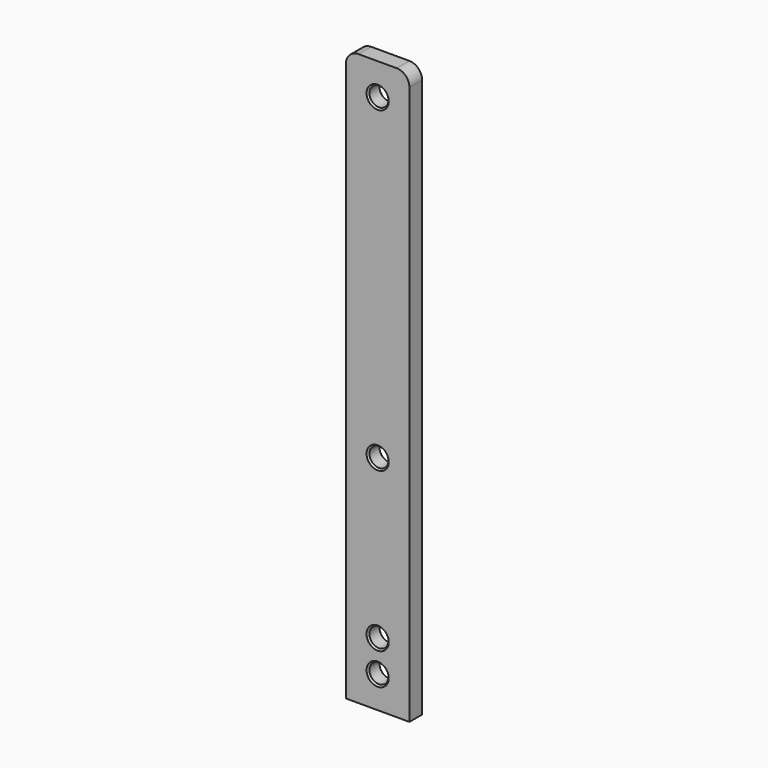
from build123d import *

# Parameters (mm, degrees)
F0_W     = 20
F0_H     = 180
F1_DEPTH = 5
F2_R     = 3
F3_DEPTH = 5.001
F5_D     = 6
F7_D     = 6
F8_SIZE  = 0.5
F9_R     = 4


with BuildPart() as f1:
    # F0 (on Front) → F1 (new body)
    with BuildSketch(Plane.XZ):
        with Locations((10, 90)):
            Rectangle(F0_W, F0_H)
    extrude(amount=F1_DEPTH)

    # F2 (on face) → F3 (cut, through all)
    with BuildSketch(Plane.XZ.offset(5)):
        with Locations((10, 170)):
            Circle(F2_R)
    extrude(amount=-F3_DEPTH, mode=Mode.SUBTRACT)

    # F5 (through all)
    with Locations(Plane.XZ.offset(5)):
        with Locations((10, 70)):
            Hole(F5_D / 2)

    # F7 (through all)
    with Locations(Plane.XZ.offset(5)):
        with Locations((10, 10), (10, 20)):
            Hole(F7_D / 2)

    # F8
    f8_edges = [f1.edges().sort_by_distance(p)[0] for p in [
        (7, -5, 170),
        (7, 0, 170),
        (7, 0, 10),
        (7, 0, 20),
        (7, 0, 70),
        (7, -5, 10),
        (7, -5, 20),
        (7, -5, 70),
    ]]
    chamfer(f8_edges, length=F8_SIZE)

    # F9
    f9_edges = [f1.edges().sort_by_distance(p)[0] for p in [
        (20, -2.5, 180),
        (0, -2.5, 180),
    ]]
    fillet(f9_edges, radius=F9_R)


solid = f1.part
